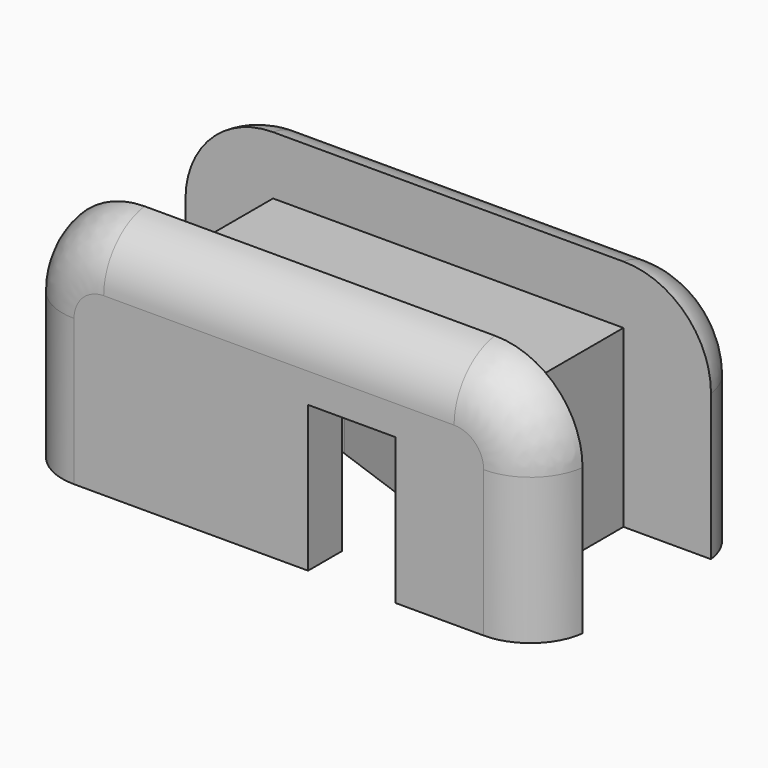
from build123d import *

# Parameters (mm, degrees)
F1_DEPTH     = 4.5
F3_DEPTH     = 2.75
F5_DEPTH     = 5
F6_T1_DEPTH  = 9.9607837082
F6_T3_DEPTH  = 12
F6_T6_ANGLE  = 90
F6_T8_ANGLE  = 90
F6_T10_ANGLE = 90
F6_T12_ANGLE = 90


# Not quite as in the source:
# - a fillet or chamfer that OpenCascade refuses, or shapes differently, is made with other operations: its cross-section is extruded or revolved along the edge and cut away or added


with BuildPart() as f1:
    # F0 (on Front) → F1 (new body, symmetric)
    with BuildSketch(Plane.XZ):
        with BuildLine():
            Line((6, 8), (-6, 8))
            ThreePointArc((-6, 8), (-8.1213203436, 7.1213203436), (-9, 5))
            Line((-9, 5), (-9, 0))
            Line((-9, 0), (9, 0))
            Line((9, 0), (9, 5))
            ThreePointArc((9, 5), (8.1213203436, 7.1213203436), (6, 8))
        make_face()
    extrude(amount=F1_DEPTH, both=True)

    # F2 (on Front) → F3 (cut, symmetric)
    with BuildSketch(Plane.XZ):
        Polygon((-24, 24), (-24, 0), (-6, 0), (-6, 6), (6, 6), (6, 0), (24, 0), (24, 24), align=None)
    extrude(amount=F3_DEPTH, both=True, mode=Mode.SUBTRACT)

    # F4 (on face) → F5 (cut)
    with BuildSketch(Plane(origin=(0, 0, 0), x_dir=(1, 0, 0), z_dir=(0, 0, -1))):
        with BuildLine():
            Line((4, -6), (4, 6))
            Line((4, 6), (1, 6))
            Line((1, 6), (1, 3.0521475958))
            Line((1, 3.0521475958), (-3.513030215, 1.4095389312))
            ThreePointArc((-3.513030215, 1.4095389312), (-4.4095389312, -0.513030215), (-2.486969785, -1.4095389312))
            Line((-2.486969785, -1.4095389312), (1, -0.1403857216))
            Line((1, -0.1403857216), (1, -6))
            Line((1, -6), (4, -6))
        make_face()
    extrude(amount=-F5_DEPTH, mode=Mode.SUBTRACT)

    # F6: fillet of radius 2 on 2 edges, made by hand

    # F6_s2 → F6_t1 (cut)
    with BuildSketch(Plane.XY.offset(-4.9607837082)):
        with BuildLine():
            ThreePointArc((9, 2.75), (8.3385621722, 4), (7.0156865167, 4.5))
            Line((7.0156865167, 4.5), (9, 4.5))
            Line((9, 4.5), (9, 2.75))
        make_face()
        with BuildLine():
            ThreePointArc((-7.0156865167, 4.5), (-8.3385621722, 4), (-9, 2.75))
            Line((-9, 2.75), (-9, 4.5))
            Line((-9, 4.5), (-7.0156865167, 4.5))
        make_face()
        with BuildLine():
            ThreePointArc((-7.0156865167, -4.5), (-8.3385621722, -4), (-9, -2.75))
            Line((-9, -2.75), (-9, -4.5))
            Line((-9, -4.5), (-7.0156865167, -4.5))
        make_face()
        with BuildLine():
            ThreePointArc((7.0156865167, -4.5), (8.3385621722, -4), (9, -2.75))
            Line((9, -2.75), (9, -4.5))
            Line((9, -4.5), (7.0156865167, -4.5))
        make_face()
    extrude(amount=F6_T1_DEPTH, mode=Mode.SUBTRACT)

    # F6_s4 → F6_t3 (cut)
    with BuildSketch(Plane.YZ.offset(-6)):
        with BuildLine():
            ThreePointArc((2.75, 8), (4, 7.3385621722), (4.5, 6.0156865167))
            Line((4.5, 6.0156865167), (4.5, 8))
            Line((4.5, 8), (2.75, 8))
        make_face()
        with BuildLine():
            ThreePointArc((-4.5, 6.0156865167), (-4, 7.3385621722), (-2.75, 8))
            Line((-2.75, 8), (-4.5, 8))
            Line((-4.5, 8), (-4.5, 6.0156865167))
        make_face()
    extrude(amount=F6_T3_DEPTH, mode=Mode.SUBTRACT)

    # F6_s5 → F6_t6 (revolve, cut)
    with BuildSketch(Plane.YZ.offset(-6)):
        with BuildLine():
            ThreePointArc((-4.5, 6.0156865167), (-4, 7.3385621722), (-2.75, 8))
            Line((-2.75, 8), (-4.5, 8))
            Line((-4.5, 8), (-4.5, 6.0156865167))
        make_face()
    revolve(axis=Axis((-6, -4.5, 5), (0, -1, 0)), revolution_arc=F6_T6_ANGLE, mode=Mode.SUBTRACT)

    # F6_s7 → F6_t8 (revolve, cut)
    with BuildSketch(Plane.XY.offset(5)):
        with BuildLine():
            ThreePointArc((9, 2.75), (8.3385621722, 4), (7.0156865167, 4.5))
            Line((7.0156865167, 4.5), (9, 4.5))
            Line((9, 4.5), (9, 2.75))
        make_face()
    revolve(axis=Axis((6, 4.5, 5), (0, -1, 0)), revolution_arc=F6_T8_ANGLE, mode=Mode.SUBTRACT)

    # F6_s9 → F6_t10 (revolve, cut)
    with BuildSketch(Plane.YZ.offset(-6)):
        with BuildLine():
            ThreePointArc((4.5, 6.0156865167), (4, 7.3385621722), (2.75, 8))
            Line((2.75, 8), (4.5, 8))
            Line((4.5, 8), (4.5, 6.0156865167))
        make_face()
    revolve(axis=Axis((-6, 4.5, 5), (0, -1, 0)), revolution_arc=F6_T10_ANGLE, mode=Mode.SUBTRACT)

    # F6_s11 → F6_t12 (revolve, cut)
    with BuildSketch(Plane.XY.offset(5)):
        with BuildLine():
            ThreePointArc((7.0156865167, -4.5), (8.3385621722, -4), (9, -2.75))
            Line((9, -2.75), (9, -4.5))
            Line((9, -4.5), (7.0156865167, -4.5))
        make_face()
    revolve(axis=Axis((6, -4.5, 5), (0, -1, 0)), revolution_arc=F6_T12_ANGLE, mode=Mode.SUBTRACT)


solid = f1.part
